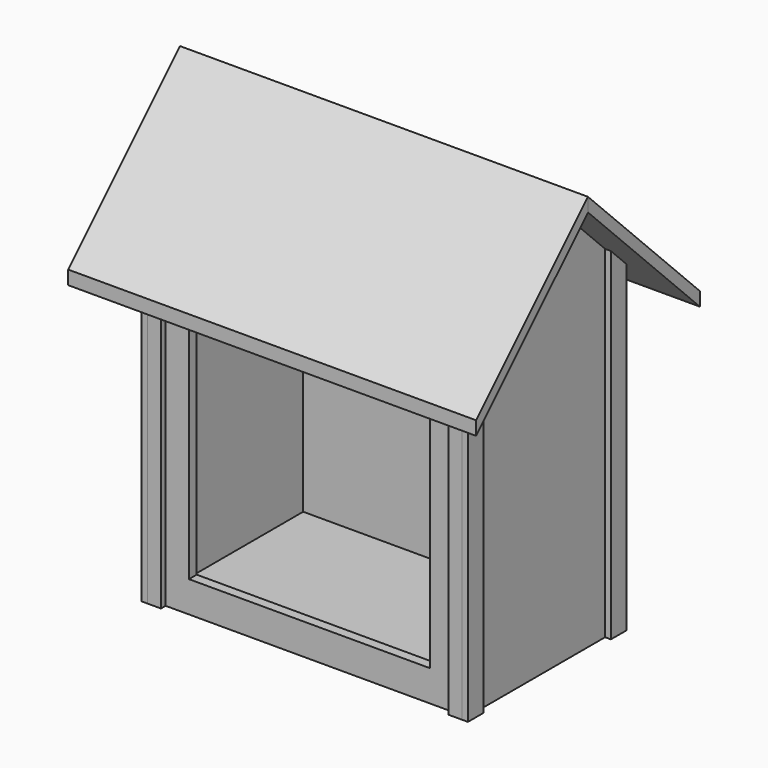
from build123d import *

# Parameters (mm, degrees)
F4_W           = 482.6
F4_H           = 273.05
F5_DEPTH       = 15.875
F6_W           = 15.875
F6_H           = 273.05
F7_DEPTH       = 688.975
F9_DEPTH       = 15.875
F12_W          = 514.35
F12_H          = 15.875
F13_DEPTH      = 552.45
F15_DEPTH      = 514.35
F16_W          = 514.35
F16_H          = 15.875
F17_DEPTH      = 552.45
F19_DEPTH      = 514.35
F20_W          = 393.7
F20_H          = 358.775
F21_DEPTH      = 15.875
F23_DEPTH      = 590.55
F23_DEPTH_BACK = 76.2
F28_DEPTH      = 9.525
F30_DEPTH      = 22.225


# Not quite as in the source:
# - a length typed as a fraction of an inch, garbled in the dataset ("3 / 203.2 mm" for 3/8 in), is restored


with BuildPart() as f5:
    # F4 (on Top) → F5 (new body)
    with BuildSketch(Plane.XY):
        with Locations((241.3, 136.525)):
            Rectangle(F4_W, F4_H)
    extrude(amount=F5_DEPTH)


with BuildPart() as f7:
    # F6 (on face) → F7 (new body)
    with BuildSketch(Plane(origin=(0, 0, 0), x_dir=(1, 0, 0), z_dir=(0, 0, -1))):
        with Locations((-7.9375, -136.525)):
            Rectangle(F6_W, F6_H)
    extrude(amount=-F7_DEPTH)

    # F8 (on face) → F9 (cut, through all)
    with BuildSketch(Plane(origin=(-15.875, 0, 0), x_dir=(0, -1, 0), z_dir=(-1, 0, 0))):
        Polygon((-273.05, 552.45), (-136.525, 688.975), (-273.05, 688.975), align=None)
        Polygon((0, 688.975), (-136.525, 688.975), (0, 552.45), align=None)
    extrude(amount=-F9_DEPTH, mode=Mode.SUBTRACT)


with BuildPart() as f11_1:
    # F11: instance of F7
    add(f7.part.mirror(Plane.YZ.offset(241.3)))


with BuildPart() as f13:
    # F12 (on face) → F13 (new body)
    with BuildSketch(Plane(origin=(0, 0, 0), x_dir=(1, 0, 0), z_dir=(0, 0, -1))):
        with Locations((241.3, -280.9875)):
            Rectangle(F12_W, F12_H)
    extrude(amount=-F13_DEPTH)

    # F14 (on face) → F15 (cut, through all)
    with BuildSketch(Plane.YZ.offset(498.475)):
        Polygon((288.925, 552.45), (273.05, 552.45), (288.925, 536.575), align=None)
    extrude(amount=-F15_DEPTH, mode=Mode.SUBTRACT)


with BuildPart() as f17:
    # F16 (on face) → F17 (new body)
    with BuildSketch(Plane(origin=(0, 0, 0), x_dir=(1, 0, 0), z_dir=(0, 0, -1))):
        with Locations((241.3, 7.9375)):
            Rectangle(F16_W, F16_H)
    extrude(amount=-F17_DEPTH)

    # F18 (on face) → F19 (cut, through all)
    with BuildSketch(Plane(origin=(-15.875, 0, 0), x_dir=(0, -1, 0), z_dir=(-1, 0, 0))):
        Polygon((15.875, 552.45), (0, 552.45), (15.875, 536.575), align=None)
    extrude(amount=-F19_DEPTH, mode=Mode.SUBTRACT)

    # F20 (on face) → F21 (cut, through all)
    with BuildSketch(Plane.XZ.offset(15.875)):
        with Locations((241.3, 230.1875)):
            Rectangle(F20_W, F20_H)
    extrude(amount=-F21_DEPTH, mode=Mode.SUBTRACT)


with BuildPart() as f23:
    # F22 (on face) → F23 (new body, two sides)
    with BuildSketch(Plane(origin=(-15.875, 0, 0), x_dir=(0, -1, 0), z_dir=(-1, 0, 0))) as f23_sk:
        Polygon((-136.525, 711.4256403027), (-136.525, 688.975), (92.075, 460.375), (92.075, 482.8256403027), align=None)
    extrude(amount=-F23_DEPTH)
    extrude(f23_sk.sketch, amount=F23_DEPTH_BACK)


with BuildPart() as f25_1:
    # F25: instance of F23
    add(f23.part.mirror(Plane.XZ.offset(-136.525)))


with BuildPart() as f28:
    # F27 (on face) → F28 (new body)
    with BuildSketch(Plane(origin=(-15.875, 0, 0), x_dir=(0, -1, 0), z_dir=(-1, 0, 0))):
        Polygon((25.4, 527.05), (-6.35, 558.8), (-6.35, 0), (25.4, 0), align=None)
    extrude(amount=F28_DEPTH)


with BuildPart() as f30:
    # F29 (on face) → F30 (new body)
    with BuildSketch(Plane.YZ.offset(-15.875)):
        Polygon((-15.875, 536.575), (-25.4, 527.05), (-25.4, 0), (-15.875, 0), align=None)
    extrude(amount=F30_DEPTH)


with BuildPart() as f31_1:
    # F31: instance of F30
    add(f30.part.mirror(Plane.XZ.offset(-136.525)))


with BuildPart() as f31_2:
    # F31: instance of F28
    add(f28.part.mirror(Plane.XZ.offset(-136.525)))


with BuildPart() as f32_1:
    # F32: instance of F28
    add(f28.part.mirror(Plane.YZ.offset(241.3)))


with BuildPart() as f32_2:
    # F32: instance of F30
    add(f30.part.mirror(Plane.YZ.offset(241.3)))


with BuildPart() as f32_3:
    # F32: instance of F31_2
    add(f31_2.part.mirror(Plane.YZ.offset(241.3)))


with BuildPart() as f32_4:
    # F32: instance of F31_1
    add(f31_1.part.mirror(Plane.YZ.offset(241.3)))


solid = Compound([f5.part, f7.part, f11_1.part, f13.part, f17.part, f23.part, f25_1.part, f28.part, f30.part, f31_1.part, f31_2.part, f32_1.part, f32_2.part, f32_3.part, f32_4.part])
